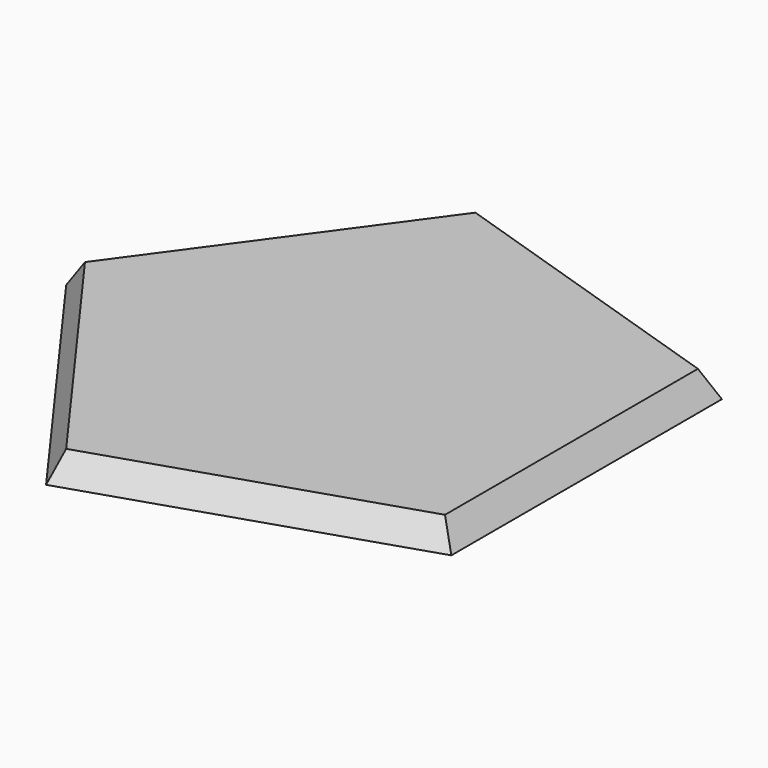
from build123d import *

# Parameters (mm, degrees)
F1_DEPTH = 14
F2_SIZE2 = 8.082894
F2_SIZE  = 13.99999


# Not quite as in the source:
# - a fillet or chamfer is up to 0.001 mm smaller than in the source, because OpenCascade refuses the exact size


with BuildPart() as f1:
    # F0 (on Top) → F1 (new body)
    with BuildSketch(Plane.XY):
        Polygon((123.8743728424, -90), (123.8743728424, 90), (-47.3158000907, 145.6230589875), (-153.1171455034, 0), (-47.3158000907, -145.6230589875), align=None)
    extrude(amount=F1_DEPTH)

    # F2 (size 14 and 8.0829037687 in the source; OpenCascade refuses exactly that, so slightly less here)
    f2_edges = [f1.edges().sort_by_distance(p)[0] for p in [
        (38.279286, -117.811529, 14),
        (123.874373, 0, 14),
        (38.279286, 117.811529, 14),
        (-100.216473, 72.811529, 14),
        (-100.216473, -72.811529, 14),
    ]]
    chamfer(f2_edges, length=F2_SIZE, length2=F2_SIZE2)


with BuildPart() as f3_1:
    # F3: copy of F1
    add(f1.part)


with BuildPart() as f5_1:
    # F5: copy of F1
    add(f1.part.moved(Location((14, 14, 14))))


solid = f1.part
